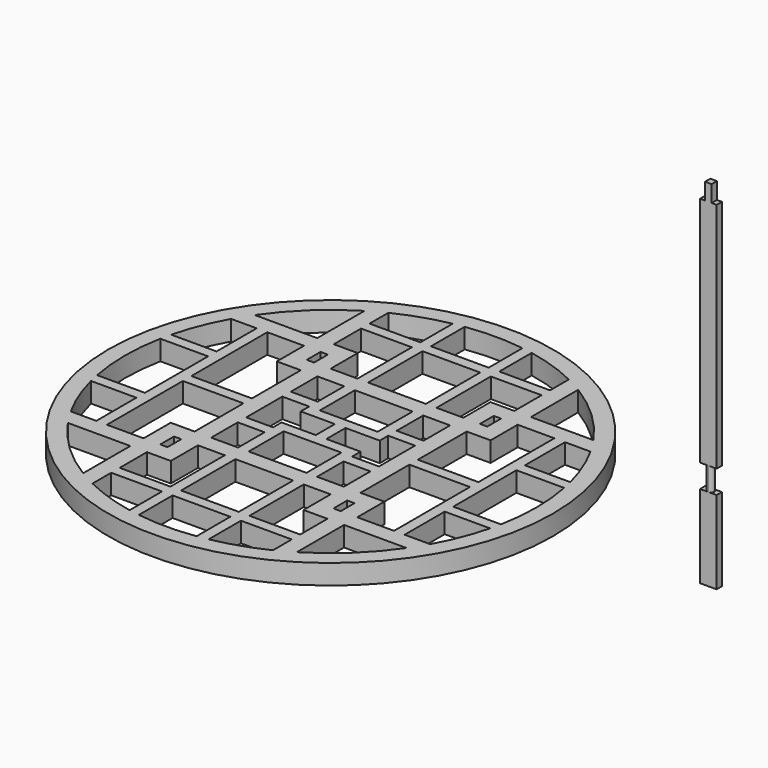
from build123d import *

# Parameters (mm, degrees)
F0_R     = 67
F0_W     = 2.2
F0_H     = 5.2
F0_W_2   = 8.1
F0_H_2   = 10
F0_W_3   = 17.4
F0_H_3   = 20.4574945033
F1_DEPTH = 6
F2_W     = 5
F2_H     = 2
F3_DEPTH = 25
F4_W     = 2
F4_H     = 2
F5_DEPTH = 7
F6_W     = 1.5
F6_H     = 2
F6_W_2   = 2
F7_DEPTH = 70
F8_W     = 2
F8_H     = 2
F9_DEPTH = 5
F10_R    = 0.99999


# Not quite as in the source:
# - a fillet or chamfer is up to 0.001 mm smaller than in the source, because OpenCascade refuses the exact size


with BuildPart() as f1:
    # F0 (on Top) → F1 (new body)
    with BuildSketch(Plane.XY):
        Circle(F0_R)
        with BuildLine():
            Line((-51.0388087635, -35.2), (-32.2, -35.2))
            Line((-32.2, -35.2), (-32.2, -52.9826386659))
            ThreePointArc((-32.2, -52.9826386659), (-42.5585523787, -45.0862464553), (-51.0388087635, -35.2))
        make_face(mode=Mode.SUBTRACT)
        with BuildLine():
            ThreePointArc((-11.9, -60.8472678105), (-19.7176969099, -58.7810550141), (-27.2, -55.7149890066))
            Line((-27.2, -55.7149890066), (-27.2, -48.6574945033))
            Line((-27.2, -48.6574945033), (-11.9, -48.6574945033))
            Line((-11.9, -48.6574945033), (-11.9, -60.8472678105))
        make_face(mode=Mode.SUBTRACT)
        Polygon((-20, -35.2), (-20, -25), (-11.9, -25), (-11.9, -45.4574945033), (-27.2, -45.4574945033), (-27.2, -35.2), align=None, mode=Mode.SUBTRACT)
        with BuildLine():
            Line((-46.4564226568, -15.1), (-46.4564226568, -30.2))
            Line((-46.4564226568, -30.2), (-54.147576123, -30.2))
            ThreePointArc((-54.147576123, -30.2), (-57.6369748417, -22.8468626095), (-60.1331023647, -15.1))
            Line((-60.1331023647, -15.1), (-46.4564226568, -15.1))
        make_face(mode=Mode.SUBTRACT)
        Polygon((-25, -20), (-32.2, -20), (-32.2, -30.2), (-43.2564226568, -30.2), (-43.2564226568, -1.6), (-25, -1.6), align=None, mode=Mode.SUBTRACT)
        with Locations((-26.1, -27.6)):
            Rectangle(F0_W, F0_H, mode=Mode.SUBTRACT)
        with Locations((-15.95, -15)):
            Rectangle(F0_W_2, F0_H_2, mode=Mode.SUBTRACT)
        with BuildLine():
            ThreePointArc((8.7, -61.3865620474), (0, -62), (-8.7, -61.3865620474))
            Line((-8.7, -61.3865620474), (-8.7, -48.6574945033))
            Line((-8.7, -48.6574945033), (8.7, -48.6574945033))
            Line((8.7, -48.6574945033), (8.7, -61.3865620474))
        make_face(mode=Mode.SUBTRACT)
        with BuildLine():
            ThreePointArc((27.2, -55.7149890066), (19.7176969099, -58.7810550141), (11.9, -60.8472678105))
            Line((11.9, -60.8472678105), (11.9, -48.6574945033))
            Line((11.9, -48.6574945033), (27.2, -48.6574945033))
            Line((27.2, -48.6574945033), (27.2, -55.7149890066))
        make_face(mode=Mode.SUBTRACT)
        with Locations((0, -35.2287472516)):
            Rectangle(F0_W_3, F0_H_3, mode=Mode.SUBTRACT)
        Polygon((11.9, -25), (20, -25), (20, -35.2), (27.2, -35.2), (27.2, -45.4574945033), (11.9, -45.4574945033), align=None, mode=Mode.SUBTRACT)
        with BuildLine():
            Line((32.2, -52.9826386659), (32.2, -35.2))
            Line((32.2, -35.2), (51.0388087635, -35.2))
            ThreePointArc((51.0388087635, -35.2), (42.5585523787, -45.0862464553), (32.2, -52.9826386659))
        make_face(mode=Mode.SUBTRACT)
        with Locations((26.1, -27.6)):
            Rectangle(F0_W, F0_H, mode=Mode.SUBTRACT)
        Polygon((8.7, -20), (-8.7, -20), (-8.7, -6.8), (0, -6.8), (8.7, -6.8), align=None, mode=Mode.SUBTRACT)
        with Locations((15.95, -15)):
            Rectangle(F0_W_2, F0_H_2, mode=Mode.SUBTRACT)
        with BuildLine():
            ThreePointArc((60.1331023647, -15.1), (57.6369748417, -22.8468626095), (54.147576123, -30.2))
            Line((54.147576123, -30.2), (46.4564226568, -30.2))
            Line((46.4564226568, -30.2), (46.4564226568, -15.1))
            Line((46.4564226568, -15.1), (60.1331023647, -15.1))
        make_face(mode=Mode.SUBTRACT)
        Polygon((32.2, -30.2), (32.2, -20), (25, -20), (25, -1.6), (43.2564226568, -1.6), (43.2564226568, -30.2), align=None, mode=Mode.SUBTRACT)
        with BuildLine():
            Line((-46.4564226568, 0), (-46.4564226568, -11.9))
            Line((-46.4564226568, -11.9), (-60.8472678105, -11.9))
            ThreePointArc((-60.8472678105, -11.9), (-62, 0), (-60.8472678105, 11.9))
            Line((-60.8472678105, 11.9), (-46.4564226568, 11.9))
            Line((-46.4564226568, 11.9), (-46.4564226568, 0))
        make_face(mode=Mode.SUBTRACT)
        Polygon((-43.2564226568, 30.2), (-32.2, 30.2), (-32.2, 20), (-25, 20), (-25, 1.6), (-43.2564226568, 1.6), align=None, mode=Mode.SUBTRACT)
        with BuildLine():
            ThreePointArc((-60.1331023647, 15.1), (-57.6369748417, 22.8468626095), (-54.147576123, 30.2))
            Line((-54.147576123, 30.2), (-46.4564226568, 30.2))
            Line((-46.4564226568, 30.2), (-46.4564226568, 15.1))
            Line((-46.4564226568, 15.1), (-60.1331023647, 15.1))
        make_face(mode=Mode.SUBTRACT)
        Polygon((-11.9226723909, -3.6), (-11.9, -6.8), (-20, -6.8), (-20, 6.8), (-11.9, 6.8), (-11.9226723909, 3.6), (-1.6, 3.6), (-1.6, 0), (-1.6, -3.6), align=None, mode=Mode.SUBTRACT)
        with Locations((-15.95, 15)):
            Rectangle(F0_W_2, F0_H_2, mode=Mode.SUBTRACT)
        with Locations((-26.1, 27.6)):
            Rectangle(F0_W, F0_H, mode=Mode.SUBTRACT)
        with BuildLine():
            Line((-32.2, 52.9826386659), (-32.2, 35.2))
            Line((-32.2, 35.2), (-51.0388087635, 35.2))
            ThreePointArc((-51.0388087635, 35.2), (-42.5585523787, 45.0862464553), (-32.2, 52.9826386659))
        make_face(mode=Mode.SUBTRACT)
        Polygon((-20, 25), (-20, 35.2), (-27.2, 35.2), (-27.2, 45.4574945033), (-11.9, 45.4574945033), (-11.9, 25), align=None, mode=Mode.SUBTRACT)
        with BuildLine():
            Line((-11.9, 48.6574945033), (-27.2, 48.6574945033))
            Line((-27.2, 48.6574945033), (-27.2, 55.7149890066))
            ThreePointArc((-27.2, 55.7149890066), (-19.7176969099, 58.7810550141), (-11.9, 60.8472678105))
            Line((-11.9, 60.8472678105), (-11.9, 48.6574945033))
        make_face(mode=Mode.SUBTRACT)
        Polygon((20, -6.8), (11.9, -6.8), (11.9226723909, -3.6), (1.6, -3.6), (1.6, 0), (1.6, 3.6), (11.9226723909, 3.6), (11.9, 6.8), (20, 6.8), align=None, mode=Mode.SUBTRACT)
        Polygon((0, 6.8), (-8.7, 6.8), (-8.7, 20), (8.7, 20), (8.7, 6.8), align=None, mode=Mode.SUBTRACT)
        with Locations((15.95, 15)):
            Rectangle(F0_W_2, F0_H_2, mode=Mode.SUBTRACT)
        with Locations((26.1, 27.6)):
            Rectangle(F0_W, F0_H, mode=Mode.SUBTRACT)
        Polygon((32.2, 20), (32.2, 30.2), (43.2564226568, 30.2), (43.2564226568, 1.6), (25, 1.6), (25, 20), align=None, mode=Mode.SUBTRACT)
        with BuildLine():
            Line((60.8472678105, -11.9), (46.4564226568, -11.9))
            Line((46.4564226568, -11.9), (46.4564226568, 0))
            Line((46.4564226568, 0), (46.4564226568, 11.9))
            Line((46.4564226568, 11.9), (60.8472678105, 11.9))
            ThreePointArc((60.8472678105, 11.9), (62, 0), (60.8472678105, -11.9))
        make_face(mode=Mode.SUBTRACT)
        with BuildLine():
            Line((60.1331023647, 15.1), (46.4564226568, 15.1))
            Line((46.4564226568, 15.1), (46.4564226568, 30.2))
            Line((46.4564226568, 30.2), (54.147576123, 30.2))
            ThreePointArc((54.147576123, 30.2), (57.6369748417, 22.8468626095), (60.1331023647, 15.1))
        make_face(mode=Mode.SUBTRACT)
        with Locations((0, 35.2287472516)):
            Rectangle(F0_W_3, F0_H_3, mode=Mode.SUBTRACT)
        Polygon((27.2, 35.2), (20, 35.2), (20, 25), (11.9, 25), (11.9, 45.4574945033), (27.2, 45.4574945033), align=None, mode=Mode.SUBTRACT)
        with BuildLine():
            Line((8.7, 61.3865620474), (8.7, 48.6574945033))
            Line((8.7, 48.6574945033), (-8.7, 48.6574945033))
            Line((-8.7, 48.6574945033), (-8.7, 61.3865620474))
            ThreePointArc((-8.7, 61.3865620474), (0, 62), (8.7, 61.3865620474))
        make_face(mode=Mode.SUBTRACT)
        with BuildLine():
            ThreePointArc((11.9, 60.8472678105), (19.7176969099, 58.7810550141), (27.2, 55.7149890066))
            Line((27.2, 55.7149890066), (27.2, 48.6574945033))
            Line((27.2, 48.6574945033), (11.9, 48.6574945033))
            Line((11.9, 48.6574945033), (11.9, 60.8472678105))
        make_face(mode=Mode.SUBTRACT)
        with BuildLine():
            Line((51.0388087635, 35.2), (32.2, 35.2))
            Line((32.2, 35.2), (32.2, 52.9826386659))
            ThreePointArc((32.2, 52.9826386659), (42.5585523787, 45.0862464553), (51.0388087635, 35.2))
        make_face(mode=Mode.SUBTRACT)
    extrude(amount=F1_DEPTH)


with BuildPart() as f3:
    # F2 (on Top) → F3 (new body)
    with BuildSketch(Plane.XY):
        with Locations((111.4652666035, 3.9335545152)):
            Rectangle(F2_W, F2_H)
    extrude(amount=F3_DEPTH)

    # F4 (on face) → F5 (join)
    with BuildSketch(Plane.XY.offset(25)):
        with Locations((111.4652666035, 3.9335545152)):
            Rectangle(F4_W, F4_H)
    extrude(amount=F5_DEPTH)

    # F6 (on face) → F7 (join)
    with BuildSketch(Plane.XY.offset(32)):
        with Locations((109.7152666035, 3.9335545152)):
            Rectangle(F6_W, F6_H)
        with Locations((111.4652666035, 3.9335545152)):
            Rectangle(F6_W_2, F6_H)
        with Locations((113.2152666035, 3.9335545152)):
            Rectangle(F6_W, F6_H)
    extrude(amount=F7_DEPTH)

    # F8 (on face) → F9 (join)
    with BuildSketch(Plane.XY.offset(102)):
        with Locations((111.4652666035, 3.9335545152)):
            Rectangle(F8_W, F8_H)
    extrude(amount=F9_DEPTH)

    # F10 (radius 1 in the source; OpenCascade refuses exactly that, so slightly less here)
    f10_edges = [f3.edges().sort_by_distance(p)[0] for p in [
        (110.465267, 4.933555, 28.5),
        (110.465267, 2.933555, 28.5),
        (112.465267, 2.933555, 28.5),
        (112.465267, 4.933555, 28.5),
    ]]
    fillet(f10_edges, radius=F10_R)


solid = Compound([f1.part, f3.part])
